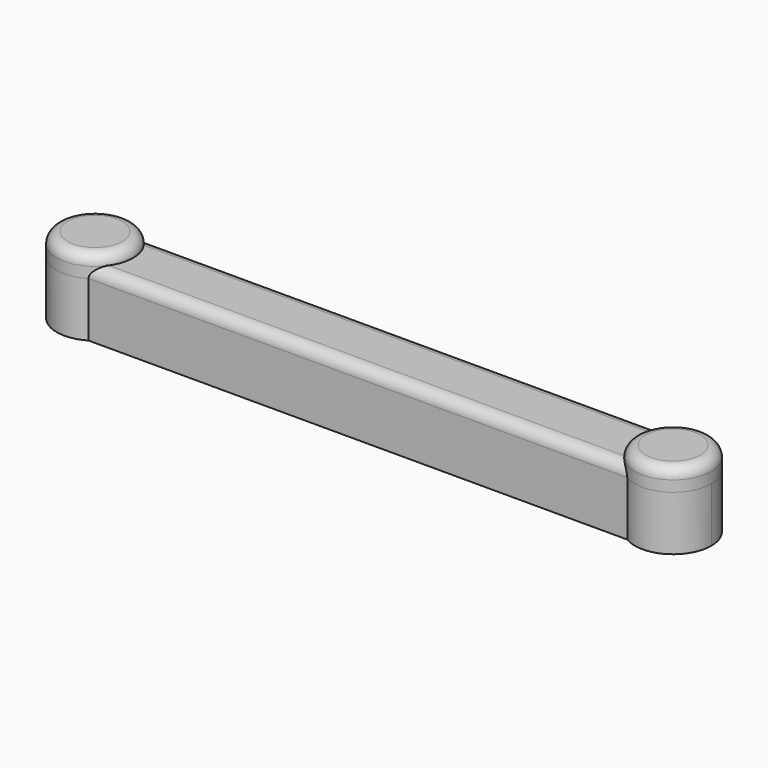
from build123d import *

# Parameters (mm, degrees)
F0_R     = 1.25
F1_DEPTH = 5
F2_DEPTH = 6
F3_R     = 3.5
F4_DEPTH = 2
F5_R     = 3.5
F6_DEPTH = 2
F7_R     = 0.99999


# Not quite as in the source:
# - a fillet or chamfer is up to 0.001 mm smaller than in the source, because OpenCascade refuses the exact size


with BuildPart() as f1:
    # F0 (on Top) → F1 (new body)
    with BuildSketch(Plane.XY):
        with BuildLine():
            ThreePointArc((-24.6972243623, -3), (-23.4537141687, -1.7234101758), (-23, 0))
            ThreePointArc((-23, 0), (-23.4537141687, 1.7234101758), (-24.6972243623, 3))
            ThreePointArc((-24.6972243623, 3), (-30, 0), (-24.6972243623, -3))
        make_face()
        with Locations((-26.5, 0)):
            Circle(F0_R, mode=Mode.SUBTRACT)
    extrude(amount=F1_DEPTH)



with BuildPart() as f1b:
    # F0 (on Top) → F1, piece 2 (new body)
    with BuildSketch(Plane.XY):
        with BuildLine():
            ThreePointArc((30, 0), (28.2234101758, 3.0462858313), (24.6972243623, 3))
            ThreePointArc((24.6972243623, 3), (23, 0), (24.6972243623, -3))
            ThreePointArc((24.6972243623, -3), (28.2234101758, -3.0462858313), (30, 0))
        make_face()
        with Locations((26.5, 0)):
            Circle(F0_R, mode=Mode.SUBTRACT)
    extrude(amount=F1_DEPTH)


with BuildPart() as f1_1:
    add(f1.part)

    add(f1b.part)  # F2 merges F1b
    # F0 (on Top) → F2 (join)
    with BuildSketch(Plane.XY):
        with BuildLine():
            ThreePointArc((-24.6972243623, 3), (-23.4537141687, 1.7234101758), (-23, 0))
            ThreePointArc((-23, 0), (-23.4537141687, -1.7234101758), (-24.6972243623, -3))
            Line((-24.6972243623, -3), (24.6972243623, -3))
            ThreePointArc((24.6972243623, -3), (23, 0), (24.6972243623, 3))
            Line((24.6972243623, 3), (-24.6972243623, 3))
        make_face()
    extrude(amount=F2_DEPTH)

    # F3 (on face) → F4 (join)
    with BuildSketch(Plane.XY.offset(5)):
        with Locations((-26.5, 0)):
            Circle(F3_R)
    extrude(amount=F4_DEPTH)

    # F5 (on face) → F6 (join)
    with BuildSketch(Plane.XY.offset(5)):
        with Locations((26.5, 0)):
            Circle(F5_R)
    extrude(amount=F6_DEPTH)

    # F7 (radius 1 in the source; OpenCascade refuses exactly that, so slightly less here)
    f7_edges = [f1_1.edges().sort_by_distance(p)[0] for p in [
        (0, 3, 6),
        (0, -3, 6),
        (23, 0, 7),
        (-30, 0, 7),
    ]]
    fillet(f7_edges, radius=F7_R)


solid = f1_1.part
